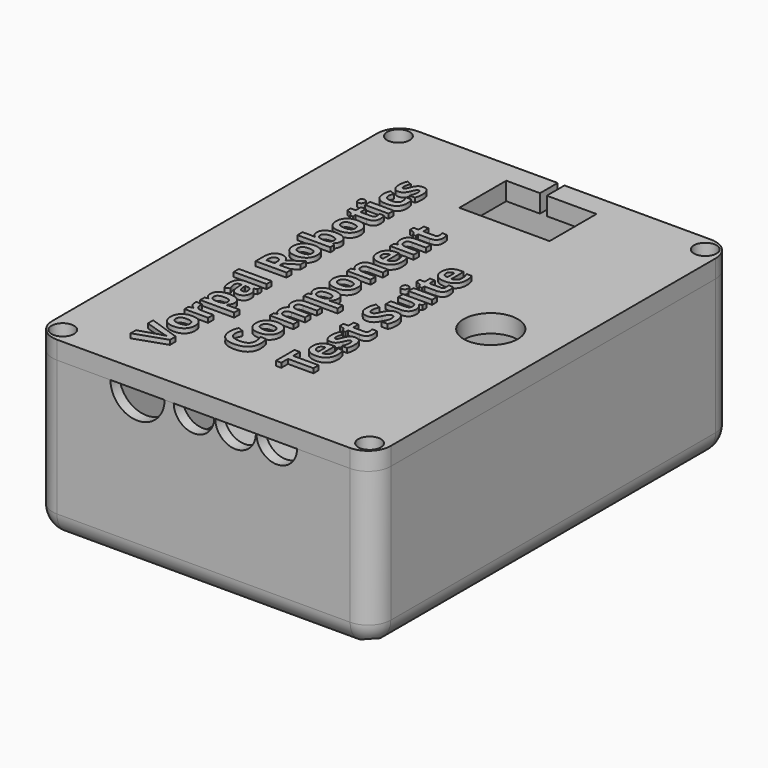
from build123d import *

# Parameters (mm, degrees)
F0_W          = 75
F0_H          = 100
F0_R          = 2.5
F0_R_2        = 1.6
F1_DEPTH      = 35
F2_T          = -2.5
F3_T1_DEPTH   = 42.5
F3_T3_DEPTH   = 65
F3_T5_DEPTH   = 90
F3_S9_W       = 5
F3_S9_H       = 5
F3_T10_DEPTH  = 5
F3_S15_W      = 5
F3_S15_H      = 5
F3_T16_DEPTH  = 5
F3_S21_W      = 5
F3_S21_H      = 5
F3_T22_DEPTH  = 5
F3_S27_W      = 5
F3_S27_H      = 5
F3_T28_DEPTH  = 5
F4_R          = 6
F4_R_2        = 4.5
F5_DEPTH      = 25
F6_DEPTH      = 4
F7_R          = 5
F8_R          = 6
F9_DEPTH      = 39.0010001
F10_TEXT_SIZE = 9.573958832
F11_DEPTH     = 1


# Not quite as in the source:
# - a fillet or chamfer that OpenCascade refuses, or shapes differently, is made with other operations: its cross-section is extruded or revolved along the edge and cut away or added
# - Text() gives the source's letters only with a copy of the font that has no kerning and outlines rounded to 1/6400 em; it was checked with that copy


with BuildPart() as f1:
    # F0 (on Top) → F1 (new body)
    with BuildSketch(Plane.XY):
        Rectangle(F0_W, F0_H)
        with Locations((-34, -46.5)):
            Circle(F0_R, mode=Mode.SUBTRACT)
        with Locations((34, -46.5)):
            Circle(F0_R, mode=Mode.SUBTRACT)
        with Locations((-34, 46.5)):
            Circle(F0_R, mode=Mode.SUBTRACT)
        with Locations((34, 46.5)):
            Circle(F0_R, mode=Mode.SUBTRACT)
        with Locations((-34, 46.5)):
            Circle(F0_R)
        with Locations((-34, 46.5)):
            Circle(F0_R_2, mode=Mode.SUBTRACT)
        with Locations((34, 46.5)):
            Circle(F0_R)
        with Locations((34, 46.5)):
            Circle(F0_R_2, mode=Mode.SUBTRACT)
        with Locations((-34, -46.5)):
            Circle(F0_R)
        with Locations((-34, -46.5)):
            Circle(F0_R_2, mode=Mode.SUBTRACT)
        with Locations((34, -46.5)):
            Circle(F0_R)
        with Locations((34, -46.5)):
            Circle(F0_R_2, mode=Mode.SUBTRACT)
    extrude(amount=-F1_DEPTH)

    # F2
    f2_openings = [f1.faces().sort_by_distance(p)[0] for p in [
        (0, 0, 0),
    ]]
    offset(amount=F2_T, openings=f2_openings)

    # F3: fillet of radius 5 on 8 edges, made by hand

    # F3_s2 → F3_t1 (cut)
    with BuildSketch(Plane.XY.offset(-30)):
        with BuildLine():
            ThreePointArc((-32.5, -50), (-36.0355339059, -48.5355339059), (-37.5, -45))
            Line((-37.5, -45), (-37.5, -50))
            Line((-37.5, -50), (-32.5, -50))
        make_face()
        with BuildLine():
            ThreePointArc((32.5, -50), (36.0355339059, -48.5355339059), (37.5, -45))
            Line((37.5, -45), (37.5, -50))
            Line((37.5, -50), (32.5, -50))
        make_face()
        with BuildLine():
            ThreePointArc((37.5, 45), (36.0355339059, 48.5355339059), (32.5, 50))
            Line((32.5, 50), (37.5, 50))
            Line((37.5, 50), (37.5, 45))
        make_face()
        with BuildLine():
            ThreePointArc((-32.5, 50), (-36.0355339059, 48.5355339059), (-37.5, 45))
            Line((-37.5, 45), (-37.5, 50))
            Line((-37.5, 50), (-32.5, 50))
        make_face()
    extrude(amount=F3_T1_DEPTH, mode=Mode.SUBTRACT)

    # F3_s4 → F3_t3 (cut)
    with BuildSketch(Plane.YZ.offset(-32.5)):
        with BuildLine():
            ThreePointArc((50, -30), (48.5355339059, -33.5355339059), (45, -35))
            Line((45, -35), (50, -35))
            Line((50, -35), (50, -30))
        make_face()
        with BuildLine():
            ThreePointArc((-50, -30), (-48.5355339059, -33.5355339059), (-45, -35))
            Line((-45, -35), (-50, -35))
            Line((-50, -35), (-50, -30))
        make_face()
    extrude(amount=F3_T3_DEPTH, mode=Mode.SUBTRACT)

    # F3_s6 → F3_t5 (cut)
    with BuildSketch(Plane.XZ.offset(-45)):
        with BuildLine():
            ThreePointArc((-37.5, -30), (-36.0355339059, -33.5355339059), (-32.5, -35))
            Line((-32.5, -35), (-37.5, -35))
            Line((-37.5, -35), (-37.5, -30))
        make_face()
        with BuildLine():
            ThreePointArc((37.5, -30), (36.0355339059, -33.5355339059), (32.5, -35))
            Line((32.5, -35), (37.5, -35))
            Line((37.5, -35), (37.5, -30))
        make_face()
    extrude(amount=F3_T5_DEPTH, mode=Mode.SUBTRACT)


with BuildPart() as f3_tool8:
    # F3_s9 → F3_t10 (new body)
    with BuildSketch(Plane.XZ.offset(45)):
        with Locations((-35, -32.5)):
            Rectangle(F3_S9_W, F3_S9_H)
    extrude(amount=F3_T10_DEPTH)

    # F3_s11 → F3_t12 (revolve, cut)
    with BuildSketch(Plane(origin=(-32.5, -45, -30), x_dir=(0.7071067812, 0, 0.7071067812), z_dir=(0.7071067812, 0, -0.7071067812))):
        with BuildLine():
            ThreePointArc((0, -5), (5, 0), (0, 5))
            Line((0, 5), (0, -5))
        make_face()
    revolve(axis=Axis((-32.5, -45, -30), (0, -1, 0)), mode=Mode.SUBTRACT)


with BuildPart() as f1_1:
    add(f1.part)

    # F3_t7: cut F3_tool8
    add(f3_tool8.part, mode=Mode.SUBTRACT)


with BuildPart() as f3_tool14:
    # F3_s15 → F3_t16 (new body)
    with BuildSketch(Plane.XZ.offset(45)):
        with Locations((35, -32.5)):
            Rectangle(F3_S15_W, F3_S15_H)
    extrude(amount=F3_T16_DEPTH)

    # F3_s17 → F3_t18 (revolve, cut)
    with BuildSketch(Plane(origin=(32.5, -45, -30), x_dir=(-0.7071067812, 0, 0.7071067812), z_dir=(0.7071067812, 0, 0.7071067812))):
        with BuildLine():
            ThreePointArc((0, -5), (5, 0), (0, 5))
            Line((0, 5), (0, -5))
        make_face()
    revolve(axis=Axis((32.5, -45, -30), (0, -1, 0)), mode=Mode.SUBTRACT)


with BuildPart() as f1_2:
    add(f1_1.part)

    # F3_t13: cut F3_tool14
    add(f3_tool14.part, mode=Mode.SUBTRACT)


with BuildPart() as f3_tool20:
    # F3_s21 → F3_t22 (new body)
    with BuildSketch(Plane.YZ.offset(32.5)):
        with Locations((47.5, -32.5)):
            Rectangle(F3_S21_W, F3_S21_H)
    extrude(amount=F3_T22_DEPTH)

    # F3_s23 → F3_t24 (revolve, cut)
    with BuildSketch(Plane(origin=(32.5, 45, -30), x_dir=(0, -0.7071067812, 0.7071067812), z_dir=(0, 0.7071067812, 0.7071067812))):
        with BuildLine():
            ThreePointArc((0, -5), (5, 0), (0, 5))
            Line((0, 5), (0, -5))
        make_face()
    revolve(axis=Axis((32.5, 45, -30), (1, 0, 0)), mode=Mode.SUBTRACT)


with BuildPart() as f1_3:
    add(f1_2.part)

    # F3_t19: cut F3_tool20
    add(f3_tool20.part, mode=Mode.SUBTRACT)


with BuildPart() as f3_tool26:
    # F3_s27 → F3_t28 (new body)
    with BuildSketch(Plane.XZ.offset(-45)):
        with Locations((-35, -32.5)):
            Rectangle(F3_S27_W, F3_S27_H)
    extrude(amount=-F3_T28_DEPTH)

    # F3_s29 → F3_t30 (revolve, cut)
    with BuildSketch(Plane(origin=(-32.5, 45, -30), x_dir=(0.7071067812, 0, 0.7071067812), z_dir=(-0.7071067812, 0, 0.7071067812))):
        with BuildLine():
            ThreePointArc((0, -5), (5, 0), (0, 5))
            Line((0, 5), (0, -5))
        make_face()
    revolve(axis=Axis((-32.5, 45, -30), (0, 1, 0)), mode=Mode.SUBTRACT)


with BuildPart() as f1_4:
    add(f1_3.part)

    # F3_t25: cut F3_tool26
    add(f3_tool26.part, mode=Mode.SUBTRACT)

    # F4 (on face) → F5 (cut)
    with BuildSketch(Plane.XZ.offset(50)):
        with Locations((-14.6300764754, 0)):
            Circle(F4_R)
        with Locations((-2.1105410997, 0.0705600396)):
            Circle(F4_R_2)
        with Locations((7.0949820802, 0)):
            Circle(F4_R_2)
        with Locations((16.2307694554, 0)):
            Circle(F4_R_2)
    extrude(amount=-F5_DEPTH, mode=Mode.SUBTRACT)


with BuildPart() as f6:
    # F0 (on Top) → F6 (new body)
    with BuildSketch(Plane.XY):
        Rectangle(F0_W, F0_H)
        with Locations((-34, -46.5)):
            Circle(F0_R, mode=Mode.SUBTRACT)
        with Locations((34, -46.5)):
            Circle(F0_R, mode=Mode.SUBTRACT)
        with Locations((-34, 46.5)):
            Circle(F0_R, mode=Mode.SUBTRACT)
        with Locations((34, 46.5)):
            Circle(F0_R, mode=Mode.SUBTRACT)
    extrude(amount=F6_DEPTH)

    # F7
    f7_edges = [f6.edges().sort_by_distance(p)[0] for p in [
        (-37.5, -50, 2),
        (37.5, -50, 2),
        (37.5, 50, 2),
        (-37.5, 50, 2),
    ]]
    fillet(f7_edges, radius=F7_R)

    # F8 (on face) → F9 (cut, through all)
    with BuildSketch(Plane.XY.offset(4)):
        Polygon((-1.5, 45.1010205144), (-8.9890961349, 45.1010205144), (-8.9890961349, 32.1010205144), (11.0109038651, 32.1010205144), (11.0109038651, 45.1010205144), (0, 45.1010205144), (0, 53.6337606609), (-1.5, 53.6337606609), align=None)
        with Locations((23.6662887037, 0)):
            Circle(F8_R)
    extrude(amount=-F9_DEPTH, mode=Mode.SUBTRACT)

    # F10 (on face) → F11 (join)
    with BuildSketch(Plane.XY.offset(4)):
        with Locations(Location((-15.9792329988, -41.6472181678), (0, 0, 90))):
            Text('Vorpal Robotics', F10_TEXT_SIZE, font='Open Sans', font_style=FontStyle.BOLD, text_align=(TextAlign.LEFT, TextAlign.BOTTOM))
        with Locations(Location((-2.9586489873, -34.184018072), (0, 0, 90))):
            Text('Component', F10_TEXT_SIZE, font='Open Sans', font_style=FontStyle.BOLD, text_align=(TextAlign.LEFT, TextAlign.BOTTOM))
        with Locations(Location((10.0619350242, -34.184018072), (0, 0, 90))):
            Text('Test Suite', F10_TEXT_SIZE, font='Open Sans', font_style=FontStyle.BOLD, text_align=(TextAlign.LEFT, TextAlign.BOTTOM))
    extrude(amount=F11_DEPTH)


solid = Compound([f1_4.part, f6.part])
